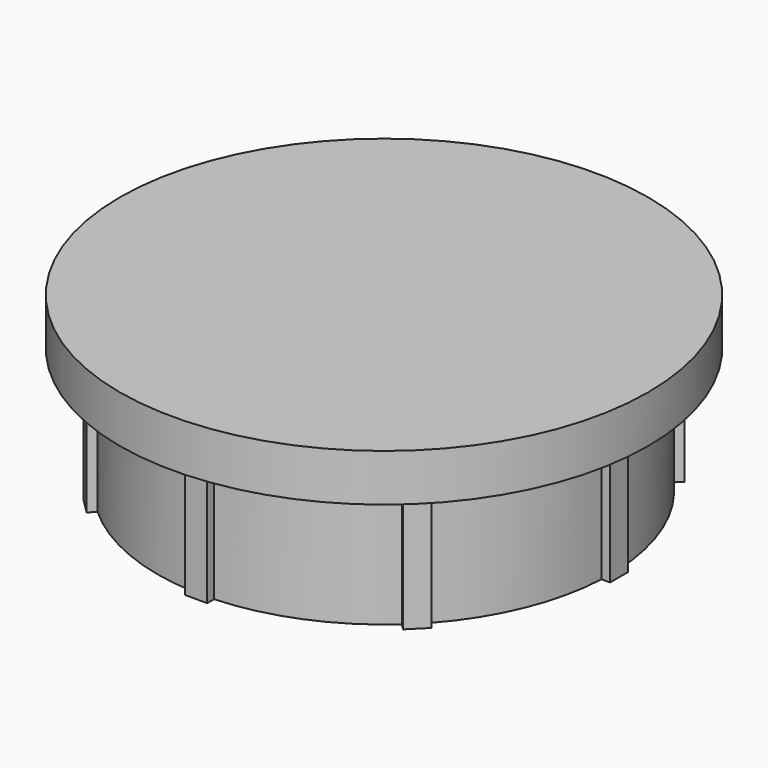
from build123d import *

# Parameters (mm, degrees)
F0_R     = 6.85
F1_DEPTH = 4.5
F2_W     = 9.5
F2_H     = 1.7
F3_ANGLE = 180


# Not quite as in the source:
# - a feature names something its author has since deleted; it is built from what else it names


with BuildPart() as f1:
    # F0 (on Top) → F1 (new body)
    with BuildSketch(Plane.XY):
        with BuildLine():
            Line((-0.4, 8.45), (-0.4, 8.1401781307))
            ThreePointArc((-0.4, 8.1401781307), (-3.1188699738, 7.52961819), (-5.4731324438, 6.0388178688))
            Line((-5.4731324438, 6.0388178688), (-5.6922095886, 6.2578950135))
            Line((-5.6922095886, 6.2578950135), (-6.2578950135, 5.6922095886))
            Line((-6.2578950135, 5.6922095886), (-6.0388178688, 5.4731324438))
            ThreePointArc((-6.0388178688, 5.4731324438), (-7.52961819, 3.1188699738), (-8.1401781307, 0.4))
            Line((-8.1401781307, 0.4), (-8.45, 0.4))
            Line((-8.45, 0.4), (-8.45, -0.4))
            Line((-8.45, -0.4), (-8.1401781307, -0.4))
            ThreePointArc((-8.1401781307, -0.4), (-7.52961819, -3.1188699738), (-6.0388178688, -5.4731324438))
            Line((-6.0388178688, -5.4731324438), (-6.2578950135, -5.6922095886))
            Line((-6.2578950135, -5.6922095886), (-5.6922095886, -6.2578950135))
            Line((-5.6922095886, -6.2578950135), (-5.4731324438, -6.0388178688))
            ThreePointArc((-5.4731324438, -6.0388178688), (-3.1188699738, -7.52961819), (-0.4, -8.1401781307))
            Line((-0.4, -8.1401781307), (-0.4, -8.45))
            Line((-0.4, -8.45), (0.4, -8.45))
            Line((0.4, -8.45), (0.4, -8.1401781307))
            ThreePointArc((0.4, -8.1401781307), (3.1188699738, -7.52961819), (5.4731324438, -6.0388178688))
            Line((5.4731324438, -6.0388178688), (5.6922095886, -6.2578950135))
            Line((5.6922095886, -6.2578950135), (6.2578950135, -5.6922095886))
            Line((6.2578950135, -5.6922095886), (6.0388178688, -5.4731324438))
            ThreePointArc((6.0388178688, -5.4731324438), (7.52961819, -3.1188699738), (8.1401781307, -0.4))
            Line((8.1401781307, -0.4), (8.45, -0.4))
            Line((8.45, -0.4), (8.45, 0.4))
            Line((8.45, 0.4), (8.1401781307, 0.4))
            ThreePointArc((8.1401781307, 0.4), (7.52961819, 3.1188699738), (6.0388178688, 5.4731324438))
            Line((6.0388178688, 5.4731324438), (6.2578950135, 5.6922095886))
            Line((6.2578950135, 5.6922095886), (5.6922095886, 6.2578950135))
            Line((5.6922095886, 6.2578950135), (5.4731324438, 6.0388178688))
            ThreePointArc((5.4731324438, 6.0388178688), (3.1188699738, 7.52961819), (0.4, 8.1401781307))
            Line((0.4, 8.1401781307), (0.4, 8.45))
            Line((0.4, 8.45), (-0.4, 8.45))
        make_face()
        Circle(F0_R, mode=Mode.SUBTRACT)
    extrude(amount=-F1_DEPTH)


with BuildPart() as f3:
    # F2 (on Front) → F3 (revolve)
    with BuildSketch(Plane.XZ):
        with Locations((-4.75, 0.85)):
            Rectangle(F2_W, F2_H)
    revolve(axis=Axis((0, 0, 0.85), (0, 0, 1)), revolution_arc=F3_ANGLE)


with BuildPart() as f4:
    # F2 (on Front) → F4 (revolve)
    with BuildSketch(Plane.XZ):
        with Locations((-4.75, 0.85)):
            Rectangle(F2_W, F2_H)
    revolve(axis=Axis((0, 0, 0.85), (0, 0, 1)))


solid = Compound([f1.part, f4.part])
